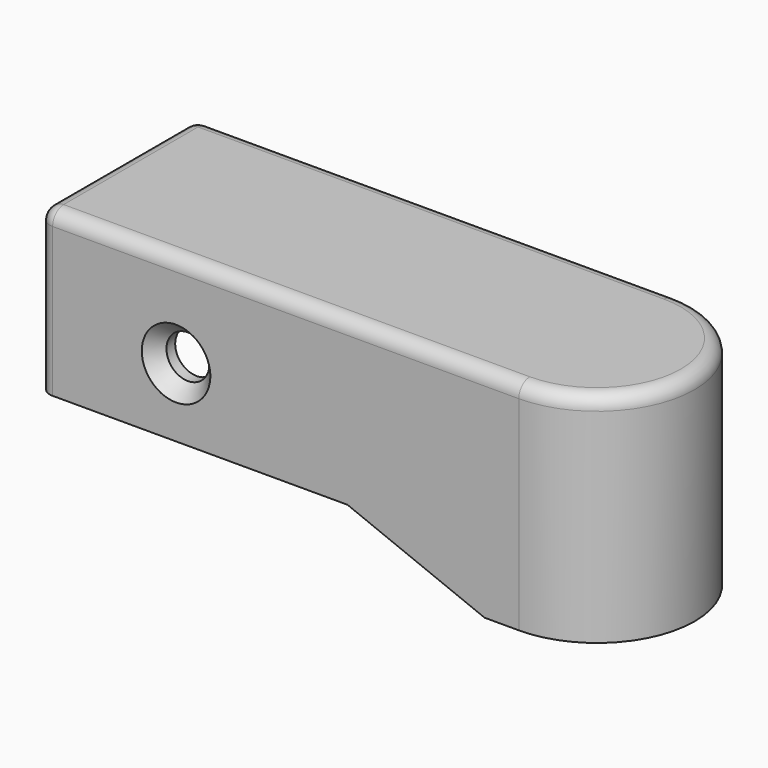
from build123d import *

# Parameters (mm, degrees)
F1_DEPTH       = 25.4
F3_DEPTH       = 4.7625
F5_D           = 7.9375
F5_DEPTH       = 12.7
F5_CSINK_D     = 12.7
F5_CSINK_ANGLE = 82
F5_TIP         = 2.3846655818
F6_R           = 2.54
F8_DEPTH       = 10.16
F9_T4_DEPTH    = 169.4252160848
F9_T9_DEPTH    = 169.4252160848


# Not quite as in the source:
# - a fillet or chamfer that OpenCascade refuses, or shapes differently, is made with other operations: its cross-section is extruded or revolved along the edge and cut away or added
# - a pattern or mirror of a feature is missing from the dataset's text; its kind, count and spacing are read off the source's solid
# - a feature names something its author has since deleted; it is built from what else it names


with BuildPart() as f1:
    # F0 (on Top) → F1 (new body)
    with BuildSketch(Plane.XY):
        with BuildLine():
            Line((38.1, 18.0975), (-50.8, 18.0975))
            Line((-50.8, 18.0975), (-50.8, 13.335))
            Line((-50.8, 13.335), (38.1, 13.335))
            ThreePointArc((38.1, 13.335), (51.435, 0), (38.1, -13.335))
            Line((38.1, -13.335), (-50.8, -13.335))
            Line((-50.8, -13.335), (-50.8, -18.0975))
            Line((-50.8, -18.0975), (38.1, -18.0975))
            ThreePointArc((38.1, -18.0975), (56.1975, 0), (38.1, 18.0975))
        make_face()
    extrude(amount=F1_DEPTH)

    # F2 (on face) → F3 (join)
    with BuildSketch(Plane.XY.offset(25.4)):
        with BuildLine():
            Line((38.1, 13.335), (-50.8, 13.335))
            Line((-50.8, 13.335), (-50.8, -13.335))
            Line((-50.8, -13.335), (38.1, -13.335))
            ThreePointArc((38.1, -13.335), (51.435, 0), (38.1, 13.335))
        make_face()
        with BuildLine():
            Line((38.1, 18.0975), (-50.8, 18.0975))
            Line((-50.8, 18.0975), (-50.8, 13.335))
            Line((-50.8, 13.335), (38.1, 13.335))
            ThreePointArc((38.1, 13.335), (51.435, 0), (38.1, -13.335))
            Line((38.1, -13.335), (-50.8, -13.335))
            Line((-50.8, -13.335), (-50.8, -18.0975))
            Line((-50.8, -18.0975), (38.1, -18.0975))
            ThreePointArc((38.1, -18.0975), (56.1975, 0), (38.1, 18.0975))
        make_face()
    extrude(amount=F3_DEPTH)

    # F5
    with Locations(Plane.XZ.offset(18.0975)):
        with Locations((-25.4, 12.7)):
            f5 = CounterSinkHole(F5_D / 2, F5_CSINK_D / 2, depth=F5_DEPTH, counter_sink_angle=F5_CSINK_ANGLE)
            with Locations((0, 0, -(F5_DEPTH + F5_TIP / 2))):  # 118° drill point
                Cone(0, F5_D / 2, F5_TIP, mode=Mode.SUBTRACT)

    # F5_copies: F5 across plane
    add(f5.mirror(Plane.ZX), mode=Mode.SUBTRACT)

    # F6
    f6_edges = [f1.edges().sort_by_distance(p)[0] for p in [
        (-50.8, 0, 30.1625),
        (-6.35, 18.0975, 30.1625),
        (-50.8, 18.0975, 15.08125),
        (56.1975, 0, 30.1625),
        (-6.35, -18.0975, 30.1625),
        (-50.8, -18.0975, 15.08125),
    ]]
    fillet(f6_edges, radius=F6_R)

    # F7 (on face) → F8 (join)
    with BuildSketch(Plane(origin=(0, 0, 0), x_dir=(1, 0, 0), z_dir=(0, 0, -1))):
        with BuildLine():
            ThreePointArc((38.1, -18.0975), (56.1975, 0), (38.1, 18.0975))
            Line((38.1, 18.0975), (0, 18.0975))
            Line((0, 18.0975), (0, 13.335))
            Line((0, 13.335), (38.1, 13.335))
            ThreePointArc((38.1, 13.335), (51.435, 0), (38.1, -13.335))
            Line((38.1, -13.335), (0, -13.335))
            Line((0, -13.335), (0, -18.0975))
            Line((0, -18.0975), (38.1, -18.0975))
        make_face()
    extrude(amount=F8_DEPTH)

    # F9: chamfer of 31.75 x 12.7 on 2 edges, made by hand


with BuildPart() as f9_tool2:
    # F9_s3 → F9_t4 (new body)
    with BuildSketch(Plane.XZ.offset(68.9963580424)):
        Polygon((31.75, -10.16), (0, 2.54), (0, -10.16), align=None)
    extrude(amount=-F9_T4_DEPTH)

    split(bisect_by=Plane.XY, keep=Keep.BOTTOM)


with BuildPart() as f1_1:
    add(f1.part)

    # F9_t1: cut F9_tool2
    add(f9_tool2.part, mode=Mode.SUBTRACT)


with BuildPart() as f9_tool7:
    # F9_s8 → F9_t9 (new body)
    with BuildSketch(Plane.XZ.offset(100.4288580424)):
        Polygon((0, 2.54), (31.75, -10.16), (0, -10.16), align=None)
    extrude(amount=-F9_T9_DEPTH)

    split(bisect_by=Plane.XY, keep=Keep.BOTTOM)


with BuildPart() as f1_2:
    add(f1_1.part)

    # F9_t6: cut F9_tool7
    add(f9_tool7.part, mode=Mode.SUBTRACT)


solid = f1_2.part
